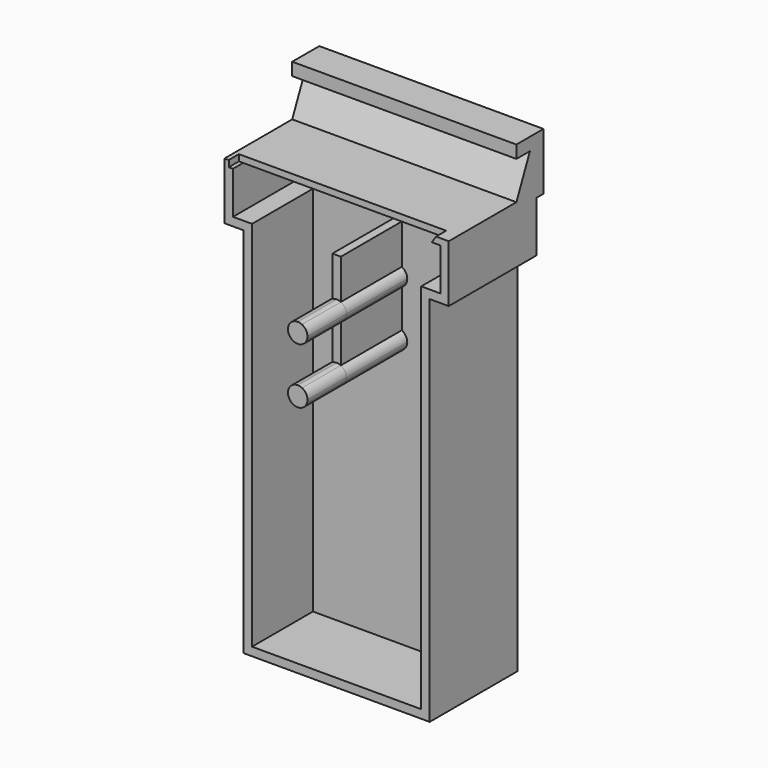
from build123d import *

# Parameters (mm, degrees)
F0_W      = 53
F0_H      = 3
F1_DEPTH  = 8
F3_DEPTH  = 53
F5_DEPTH  = 8
F6_DEPTH  = 17
F7_DEPTH  = 20
F8_W      = 1
F8_H      = 1.5
F9_DEPTH  = 8
F10_DEPTH = 20
F11_DEPTH = 17
F12_W     = 2
F12_H     = 13
F13_DEPTH = 12
F14_W     = 18
F14_H     = 2
F15_DEPTH = 2.5
F16_DEPTH = 8
F17_DEPTH = 17
F18_W     = 2
F18_H     = 18
F19_DEPTH = 2
F20_DEPTH = 88
F21_W     = 2
F21_H     = 13
F22_DEPTH = 12
F23_W     = 18
F23_H     = 2
F24_DEPTH = 4.5
F25_W     = 2
F25_H     = 18
F26_DEPTH = 88
F27_W     = 2
F27_H     = 12
F28_DEPTH = 5
F29_W     = 2
F29_H     = 12
F30_DEPTH = 5
F31_W     = 40
F31_H     = 88
F31_H_2   = 2
F32_DEPTH = 8
F34_DEPTH = 18
F35_DEPTH = 26
F36_DEPTH = 4
F37_DEPTH = 11.5
F38_W     = 40
F38_H     = 2
F39_DEPTH = 18


# Not quite as in the source:
# - a feature names something its author has since deleted; it is built from what else it names


with BuildPart() as f1:
    # F0 (on Front) → F1 (new body)
    with BuildSketch(Plane.XZ):
        with Locations((26.5, 1.5)):
            Rectangle(F0_W, F0_H)
    extrude(amount=F1_DEPTH)

    # F2 (on face) → F3 (join)
    with BuildSketch(Plane.YZ.offset(53)):
        Polygon((0, -9), (0, 0), (-4, 0), (-8, -9), align=None)
    extrude(amount=-F3_DEPTH)

    # F4 (on face) → F5 (join)
    with BuildSketch(Plane.XZ.offset(8)):
        Polygon((53, -10), (53, -9), (50, -9), (49.5, -9.75), (49, -10.5), (50, -10.5), (53, -10.5), align=None)
    extrude(amount=-F5_DEPTH)

    # F4 (on face) → F6 (join)
    with BuildSketch(Plane.XZ.offset(8)):
        Polygon((53, -10), (53, -9), (50, -9), (49.5, -9.75), (49, -10.5), (50, -10.5), (53, -10.5), align=None)
    extrude(amount=F6_DEPTH)

    # F4 (on face) → F7 (join)
    with BuildSketch(Plane.XZ.offset(8)):
        Polygon((53, -10), (53, -9), (50, -9), (49.5, -9.75), (49, -10.5), (50, -10.5), (53, -10.5), align=None)
    extrude(amount=F7_DEPTH)

    # F8 (on face) → F9 (join)
    with BuildSketch(Plane.XZ.offset(8)):
        with Locations((0.5, -9.75)):
            Rectangle(F8_W, F8_H)
        Polygon((8, -9), (1, -9), (1, -10.5), (8, -10.5), (49.5, -10.5), (49.5, -9), align=None)
    extrude(amount=-F9_DEPTH)

    # F8 (on face) → F10 (join)
    with BuildSketch(Plane.XZ.offset(8)):
        with Locations((0.5, -9.75)):
            Rectangle(F8_W, F8_H)
    extrude(amount=F10_DEPTH)

    # F8 (on face) → F11 (join)
    with BuildSketch(Plane.XZ.offset(8)):
        Polygon((8, -9), (1, -9), (1, -10.5), (8, -10.5), (49.5, -10.5), (49.5, -9), align=None)
    extrude(amount=F11_DEPTH)

    # F12 (on face) → F13 (join)
    with BuildSketch(Plane(origin=(0, 0, -10.5), x_dir=(1, 0, 0), z_dir=(0, 0, -1))):
        with Locations((52, 21.5)):
            Rectangle(F12_W, F12_H)
    extrude(amount=F13_DEPTH)

    # F14 (on face) → F15 (join)
    with BuildSketch(Plane(origin=(51, 0, 0), x_dir=(0, -1, 0), z_dir=(-1, 0, 0))):
        with Locations((19, -21.5)):
            Rectangle(F14_W, F14_H)
    extrude(amount=F15_DEPTH)

    # F4 (on face) → F16 (join)
    with BuildSketch(Plane.XZ.offset(8)):
        Polygon((49.5, -9.75), (50, -9), (49.5, -9), align=None)
    extrude(amount=-F16_DEPTH)

    # F4 (on face) → F17 (join)
    with BuildSketch(Plane.XZ.offset(8)):
        Polygon((49.5, -9.75), (50, -9), (49.5, -9), align=None)
    extrude(amount=F17_DEPTH)

    # F18 (on face) → F19 (join)
    with BuildSketch(Plane(origin=(0, 0, -22.5), x_dir=(1, 0, 0), z_dir=(0, 0, -1))):
        with Locations((47.5, 19)):
            Rectangle(F18_W, F18_H)
    extrude(amount=-F19_DEPTH)

    # F18 (on face) → F20 (join)
    with BuildSketch(Plane(origin=(0, 0, -22.5), x_dir=(1, 0, 0), z_dir=(0, 0, -1))):
        with Locations((47.5, 19)):
            Rectangle(F18_W, F18_H)
    extrude(amount=F20_DEPTH)

    # F21 (on face) → F22 (join)
    with BuildSketch(Plane(origin=(0, 0, -10.5), x_dir=(1, 0, 0), z_dir=(0, 0, -1))):
        with Locations((1, 21.5)):
            Rectangle(F21_W, F21_H)
    extrude(amount=F22_DEPTH)

    # F23 (on face) → F24 (join)
    with BuildSketch(Plane.YZ.offset(2)):
        with Locations((-19, -21.5)):
            Rectangle(F23_W, F23_H)
    extrude(amount=F24_DEPTH)

    # F25 (on face) → F26 (join)
    with BuildSketch(Plane(origin=(0, 0, -22.5), x_dir=(1, 0, 0), z_dir=(0, 0, -1))):
        with Locations((5.5, 19)):
            Rectangle(F25_W, F25_H)
    extrude(amount=F26_DEPTH)

    # F27 (on face) → F28 (join)
    with BuildSketch(Plane(origin=(0, -15, 0), x_dir=(-1, 0, 0), z_dir=(0, 1, 0))):
        with Locations((-1, -16.5)):
            Rectangle(F27_W, F27_H)
    extrude(amount=F28_DEPTH)

    # F29 (on face) → F30 (join)
    with BuildSketch(Plane(origin=(0, -15, 0), x_dir=(-1, 0, 0), z_dir=(0, 1, 0))):
        with Locations((-52, -16.5)):
            Rectangle(F29_W, F29_H)
    extrude(amount=F30_DEPTH)

    # F30_face (on face) + F31 (on face) → F32 (join)
    with BuildSketch(Plane(origin=(48.0705741627, -10, -58.8205741627), x_dir=(-1, 0, 0), z_dir=(0, 1, 0))):
        Polygon((-2.9294258373, 38.3205741627), (-2.9294258373, 48.3205741627), (-4.9294258373, 48.3205741627), (-4.9294258373, 36.3205741627), (-0.4294258373, 36.3205741627), (-0.4294258373, -51.6794258373), (1.5705741627, -51.6794258373), (1.5705741627, 38.3205741627), align=None)
    with BuildSketch(Plane(origin=(0, -10, 0), x_dir=(-1, 0, 0), z_dir=(0, 1, 0))):
        Polygon((-2, -20.5), (-2, -10.5), (-51, -10.5), (-51, -20.5), (-46.5, -20.5), (-6.5, -20.5), align=None)
        Polygon((0, -10.5), (-2, -10.5), (-2, -20.5), (-6.5, -20.5), (-6.5, -108.5), (-6.5, -110.5), (-4.5, -110.5), (-4.5, -22.5), (0, -22.5), align=None)
        with Locations((-26.5, -64.5)):
            Rectangle(F31_W, F31_H)
        with Locations((-26.5, -109.5)):
            Rectangle(F31_W, F31_H_2)
    extrude(amount=F32_DEPTH)

    # F33 (on face) → F34 (join)
    with BuildSketch(Plane.XZ.offset(28)):
        with BuildLine():
            ThreePointArc((26.5, -42.9), (25.9870830919, -42.9579214453), (25.5, -43.1287684823))
            Line((25.5, -43.1287684823), (25.5, -47.2712315177))
            ThreePointArc((25.5, -47.2712315177), (25.9870830919, -47.4420785547), (26.5, -47.5))
            Line((26.5, -47.5), (26.5, -42.9))
        make_face()
        with BuildLine():
            ThreePointArc((27.5, -43.1287684823), (27.0129169081, -42.9579214453), (26.5, -42.9))
            Line((26.5, -42.9), (26.5, -47.5))
            ThreePointArc((26.5, -47.5), (27.0129169081, -47.4420785547), (27.5, -47.2712315177))
            Line((27.5, -47.2712315177), (27.5, -43.1287684823))
        make_face()
        with BuildLine():
            ThreePointArc((27.5, -34.0712315177), (27.0129169081, -34.2420785547), (26.5, -34.3))
            Line((26.5, -34.3), (26.5, -42.9))
            ThreePointArc((26.5, -42.9), (27.0129169081, -42.9579214453), (27.5, -43.1287684823))
            Line((27.5, -43.1287684823), (27.5, -34.0712315177))
        make_face()
        with BuildLine():
            ThreePointArc((26.5, -34.3), (25.9870830919, -34.2420785547), (25.5, -34.0712315177))
            Line((25.5, -34.0712315177), (25.5, -43.1287684823))
            ThreePointArc((25.5, -43.1287684823), (25.9870830919, -42.9579214453), (26.5, -42.9))
            Line((26.5, -42.9), (26.5, -34.3))
        make_face()
        with BuildLine():
            ThreePointArc((26.5, -29.7), (25.9870830919, -29.7579214453), (25.5, -29.9287684823))
            Line((25.5, -29.9287684823), (25.5, -34.0712315177))
            ThreePointArc((25.5, -34.0712315177), (25.9870830919, -34.2420785547), (26.5, -34.3))
            Line((26.5, -34.3), (26.5, -29.7))
        make_face()
        with BuildLine():
            ThreePointArc((27.5, -29.9287684823), (27.0129169081, -29.7579214453), (26.5, -29.7))
            Line((26.5, -29.7), (26.5, -34.3))
            ThreePointArc((26.5, -34.3), (27.0129169081, -34.2420785547), (27.5, -34.0712315177))
            Line((27.5, -34.0712315177), (27.5, -29.9287684823))
        make_face()
        with BuildLine():
            Line((27.5, -20.5), (26.5, -20.5))
            Line((26.5, -20.5), (26.5, -29.7))
            ThreePointArc((26.5, -29.7), (27.0129169081, -29.7579214453), (27.5, -29.9287684823))
            Line((27.5, -29.9287684823), (27.5, -20.5))
        make_face()
        with BuildLine():
            Line((26.5, -20.5), (25.5, -20.5))
            Line((25.5, -20.5), (25.5, -29.9287684823))
            ThreePointArc((25.5, -29.9287684823), (25.9870830919, -29.7579214453), (26.5, -29.7))
            Line((26.5, -29.7), (26.5, -20.5))
        make_face()
    extrude(amount=-F34_DEPTH)

    # F33 (on face) → F35 (join)
    with BuildSketch(Plane.XZ.offset(28)):
        with BuildLine():
            ThreePointArc((28.8, -32), (28.4480759739, -30.7772980739), (27.5, -29.9287684823))
            Line((27.5, -29.9287684823), (27.5, -34.0712315177))
            ThreePointArc((27.5, -34.0712315177), (28.4480759739, -33.2227019261), (28.8, -32))
        make_face()
        with BuildLine():
            ThreePointArc((27.5, -29.9287684823), (27.0129169081, -29.7579214453), (26.5, -29.7))
            Line((26.5, -29.7), (26.5, -34.3))
            ThreePointArc((26.5, -34.3), (27.0129169081, -34.2420785547), (27.5, -34.0712315177))
            Line((27.5, -34.0712315177), (27.5, -29.9287684823))
        make_face()
        with BuildLine():
            ThreePointArc((26.5, -29.7), (25.9870830919, -29.7579214453), (25.5, -29.9287684823))
            Line((25.5, -29.9287684823), (25.5, -34.0712315177))
            ThreePointArc((25.5, -34.0712315177), (25.9870830919, -34.2420785547), (26.5, -34.3))
            Line((26.5, -34.3), (26.5, -29.7))
        make_face()
        with BuildLine():
            Line((25.5, -34.0712315177), (25.5, -29.9287684823))
            ThreePointArc((25.5, -29.9287684823), (24.2, -32), (25.5, -34.0712315177))
        make_face()
        with BuildLine():
            ThreePointArc((26.5, -42.9), (25.9870830919, -42.9579214453), (25.5, -43.1287684823))
            Line((25.5, -43.1287684823), (25.5, -47.2712315177))
            ThreePointArc((25.5, -47.2712315177), (25.9870830919, -47.4420785547), (26.5, -47.5))
            Line((26.5, -47.5), (26.5, -42.9))
        make_face()
        with BuildLine():
            Line((25.5, -47.2712315177), (25.5, -43.1287684823))
            ThreePointArc((25.5, -43.1287684823), (24.2, -45.2), (25.5, -47.2712315177))
        make_face()
        with BuildLine():
            ThreePointArc((27.5, -43.1287684823), (27.0129169081, -42.9579214453), (26.5, -42.9))
            Line((26.5, -42.9), (26.5, -47.5))
            ThreePointArc((26.5, -47.5), (27.0129169081, -47.4420785547), (27.5, -47.2712315177))
            Line((27.5, -47.2712315177), (27.5, -43.1287684823))
        make_face()
        with BuildLine():
            ThreePointArc((28.8, -45.2), (28.4480759739, -43.9772980739), (27.5, -43.1287684823))
            Line((27.5, -43.1287684823), (27.5, -47.2712315177))
            ThreePointArc((27.5, -47.2712315177), (28.4480759739, -46.4227019261), (28.8, -45.2))
        make_face()
    extrude(amount=-F35_DEPTH)

    # F33 (on face) → F36 (cut)
    with BuildSketch(Plane.XZ.offset(28)):
        with BuildLine():
            Line((27.5, -20.5), (26.5, -20.5))
            Line((26.5, -20.5), (26.5, -29.7))
            ThreePointArc((26.5, -29.7), (27.0129169081, -29.7579214453), (27.5, -29.9287684823))
            Line((27.5, -29.9287684823), (27.5, -20.5))
        make_face()
        with BuildLine():
            Line((26.5, -20.5), (25.5, -20.5))
            Line((25.5, -20.5), (25.5, -29.9287684823))
            ThreePointArc((25.5, -29.9287684823), (25.9870830919, -29.7579214453), (26.5, -29.7))
            Line((26.5, -29.7), (26.5, -20.5))
        make_face()
        with BuildLine():
            ThreePointArc((26.5, -29.7), (25.9870830919, -29.7579214453), (25.5, -29.9287684823))
            Line((25.5, -29.9287684823), (25.5, -34.0712315177))
            ThreePointArc((25.5, -34.0712315177), (25.9870830919, -34.2420785547), (26.5, -34.3))
            Line((26.5, -34.3), (26.5, -29.7))
        make_face()
        with BuildLine():
            ThreePointArc((27.5, -29.9287684823), (27.0129169081, -29.7579214453), (26.5, -29.7))
            Line((26.5, -29.7), (26.5, -34.3))
            ThreePointArc((26.5, -34.3), (27.0129169081, -34.2420785547), (27.5, -34.0712315177))
            Line((27.5, -34.0712315177), (27.5, -29.9287684823))
        make_face()
        with BuildLine():
            ThreePointArc((27.5, -34.0712315177), (27.0129169081, -34.2420785547), (26.5, -34.3))
            Line((26.5, -34.3), (26.5, -42.9))
            ThreePointArc((26.5, -42.9), (27.0129169081, -42.9579214453), (27.5, -43.1287684823))
            Line((27.5, -43.1287684823), (27.5, -34.0712315177))
        make_face()
        with BuildLine():
            ThreePointArc((26.5, -34.3), (25.9870830919, -34.2420785547), (25.5, -34.0712315177))
            Line((25.5, -34.0712315177), (25.5, -43.1287684823))
            ThreePointArc((25.5, -43.1287684823), (25.9870830919, -42.9579214453), (26.5, -42.9))
            Line((26.5, -42.9), (26.5, -34.3))
        make_face()
        with BuildLine():
            ThreePointArc((26.5, -42.9), (25.9870830919, -42.9579214453), (25.5, -43.1287684823))
            Line((25.5, -43.1287684823), (25.5, -47.2712315177))
            ThreePointArc((25.5, -47.2712315177), (25.9870830919, -47.4420785547), (26.5, -47.5))
            Line((26.5, -47.5), (26.5, -42.9))
        make_face()
        with BuildLine():
            ThreePointArc((27.5, -43.1287684823), (27.0129169081, -42.9579214453), (26.5, -42.9))
            Line((26.5, -42.9), (26.5, -47.5))
            ThreePointArc((26.5, -47.5), (27.0129169081, -47.4420785547), (27.5, -47.2712315177))
            Line((27.5, -47.2712315177), (27.5, -43.1287684823))
        make_face()
    extrude(amount=F36_DEPTH, mode=Mode.SUBTRACT)

    # F33 (on face) → F37 (join)
    with BuildSketch(Plane.XZ.offset(28)):
        with BuildLine():
            ThreePointArc((28.8, -32), (28.4480759739, -30.7772980739), (27.5, -29.9287684823))
            Line((27.5, -29.9287684823), (27.5, -34.0712315177))
            ThreePointArc((27.5, -34.0712315177), (28.4480759739, -33.2227019261), (28.8, -32))
        make_face()
        with BuildLine():
            ThreePointArc((27.5, -29.9287684823), (27.0129169081, -29.7579214453), (26.5, -29.7))
            Line((26.5, -29.7), (26.5, -34.3))
            ThreePointArc((26.5, -34.3), (27.0129169081, -34.2420785547), (27.5, -34.0712315177))
            Line((27.5, -34.0712315177), (27.5, -29.9287684823))
        make_face()
        with BuildLine():
            ThreePointArc((26.5, -29.7), (25.9870830919, -29.7579214453), (25.5, -29.9287684823))
            Line((25.5, -29.9287684823), (25.5, -34.0712315177))
            ThreePointArc((25.5, -34.0712315177), (25.9870830919, -34.2420785547), (26.5, -34.3))
            Line((26.5, -34.3), (26.5, -29.7))
        make_face()
        with BuildLine():
            Line((25.5, -34.0712315177), (25.5, -29.9287684823))
            ThreePointArc((25.5, -29.9287684823), (24.2, -32), (25.5, -34.0712315177))
        make_face()
        with BuildLine():
            Line((25.5, -47.2712315177), (25.5, -43.1287684823))
            ThreePointArc((25.5, -43.1287684823), (24.2, -45.2), (25.5, -47.2712315177))
        make_face()
        with BuildLine():
            ThreePointArc((26.5, -42.9), (25.9870830919, -42.9579214453), (25.5, -43.1287684823))
            Line((25.5, -43.1287684823), (25.5, -47.2712315177))
            ThreePointArc((25.5, -47.2712315177), (25.9870830919, -47.4420785547), (26.5, -47.5))
            Line((26.5, -47.5), (26.5, -42.9))
        make_face()
        with BuildLine():
            ThreePointArc((27.5, -43.1287684823), (27.0129169081, -42.9579214453), (26.5, -42.9))
            Line((26.5, -42.9), (26.5, -47.5))
            ThreePointArc((26.5, -47.5), (27.0129169081, -47.4420785547), (27.5, -47.2712315177))
            Line((27.5, -47.2712315177), (27.5, -43.1287684823))
        make_face()
        with BuildLine():
            ThreePointArc((28.8, -45.2), (28.4480759739, -43.9772980739), (27.5, -43.1287684823))
            Line((27.5, -43.1287684823), (27.5, -47.2712315177))
            ThreePointArc((27.5, -47.2712315177), (28.4480759739, -46.4227019261), (28.8, -45.2))
        make_face()
    extrude(amount=F37_DEPTH)

    # F38 (on face) → F39 (join)
    with BuildSketch(Plane.XZ.offset(10)):
        with Locations((26.5, -109.5)):
            Rectangle(F38_W, F38_H)
    extrude(amount=F39_DEPTH)


solid = f1.part
